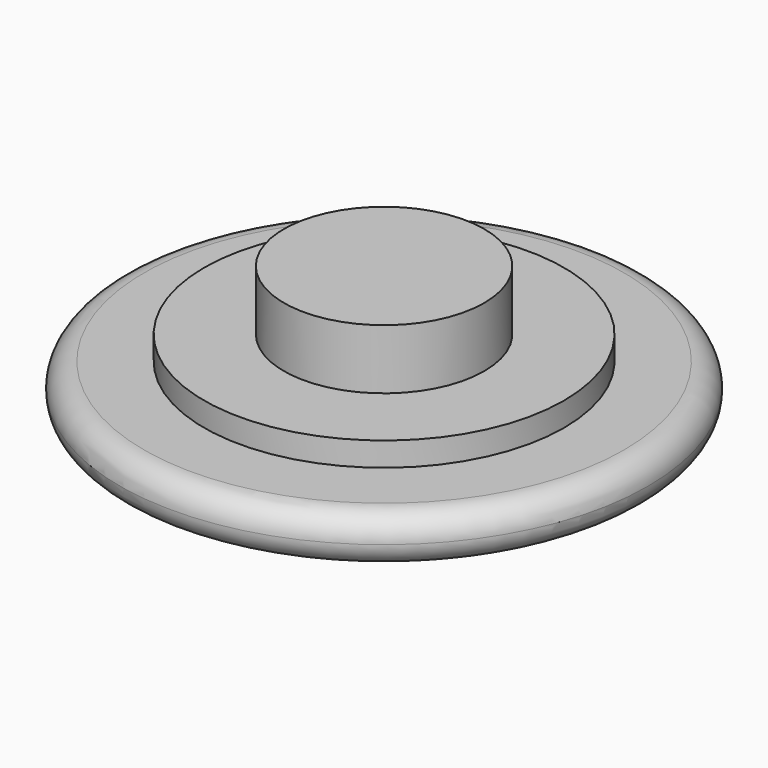
from build123d import *

# Parameters (mm, degrees)
F0_R         = 11
F0_R_2       = 7.5
F1_DEPTH     = 2
F0_R_3       = 4.175
F2_DEPTH     = 3
F3_DEPTH     = 5.5
F4_R         = 0.99999
F5_TEXT_SIZE = 4.0022763033
F6_DEPTH     = 1


# Not quite as in the source:
# - a fillet or chamfer is up to 0.001 mm smaller than in the source, because OpenCascade refuses the exact size
# - Text() gives the source's letters only with a copy of the font that has no kerning and outlines rounded to 1/6400 em; it was checked with that copy


with BuildPart() as f1:
    # F0 (on Top) → F1 (new body)
    with BuildSketch(Plane.XY):
        Circle(F0_R)
        Circle(F0_R_2, mode=Mode.SUBTRACT)
    extrude(amount=F1_DEPTH)

    # F0 (on Top) → F2 (join)
    with BuildSketch(Plane.XY):
        Circle(F0_R_2)
        Circle(F0_R_3, mode=Mode.SUBTRACT)
    extrude(amount=F2_DEPTH)

    # F0 (on Top) → F3 (join)
    with BuildSketch(Plane.XY):
        Circle(F0_R_3)
    extrude(amount=F3_DEPTH)

    # F4 (radius 1 in the source; OpenCascade refuses exactly that, so slightly less here)
    f4_edges = [f1.edges().sort_by_distance(p)[0] for p in [
        (-11, 0, 2),
        (-11, 0, 0),
    ]]
    fillet(f4_edges, radius=F4_R)

    # F5 (on face) → F6 (cut)
    with BuildSketch(Plane(origin=(0, 0, 0), x_dir=(1, 0, 0), z_dir=(0, 0, -1))):
        with Locations((-9.8921504982, -1.4647042438)):
            Text('LTD Alyssa', F5_TEXT_SIZE, font='Open Sans', text_align=(TextAlign.LEFT, TextAlign.BOTTOM))
    extrude(amount=-F6_DEPTH, mode=Mode.SUBTRACT)


solid = f1.part
